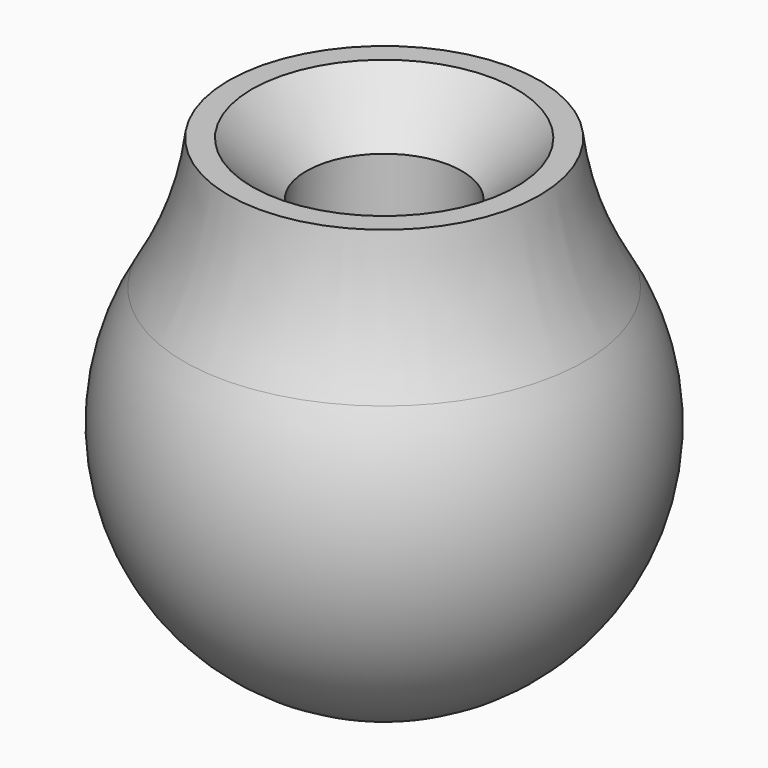
from build123d import *

# Parameters (mm, degrees)
F2_SIZE = 1.4


# Not quite as in the source:
# - a fillet or chamfer that OpenCascade refuses, or shapes differently, is made with other operations: its cross-section is extruded or revolved along the edge and cut away or added


with BuildPart() as f1:
    # F0 (on Front) → F1 (revolve)
    with BuildSketch(Plane.XZ):
        with BuildLine():
            ThreePointArc((0, 0), (-3.8637033052, 2.9647238196), (-2, 7.4641016151))
            Line((-2, 7.4641016151), (-2, 10.4641016151))
            Line((-2, 10.4641016151), (-4, 10.4641016151))
            Line((-4, 10.4641016151), (-4, 8.472135955))
            ThreePointArc((-4, 8.472135955), (-5.6050341538, 1.8590674614), (0, -2))
            Line((0, -2), (0, 0))
        make_face()
    revolve(axis=Axis((0, 0, -1), (0, 0, -1)))

    # F2
    f2_edges = [f1.edges().sort_by_distance(p)[0] for p in [
        (2, 0, 10.464102),
    ]]
    chamfer(f2_edges, length=F2_SIZE)

    # F3: fillet of radius 8.5913249715 on 1 edges, made by hand

    # F3_s1 → F3_t2 (revolve)
    with BuildSketch(Plane.XZ):
        with BuildLine():
            ThreePointArc((-4, 10.4641016151), (-4.397901087, 8.7079815946), (-5.1530970812, 7.0733679363))
            ThreePointArc((-5.1530970812, 7.0733679363), (-4.6296797445, 7.8165515145), (-4, 8.472135955))
            Line((-4, 8.472135955), (-4, 10.4641016151))
        make_face()
    revolve(axis=Axis((0, 0, 8.472135955), (0, 0, -1)))


solid = f1.part
